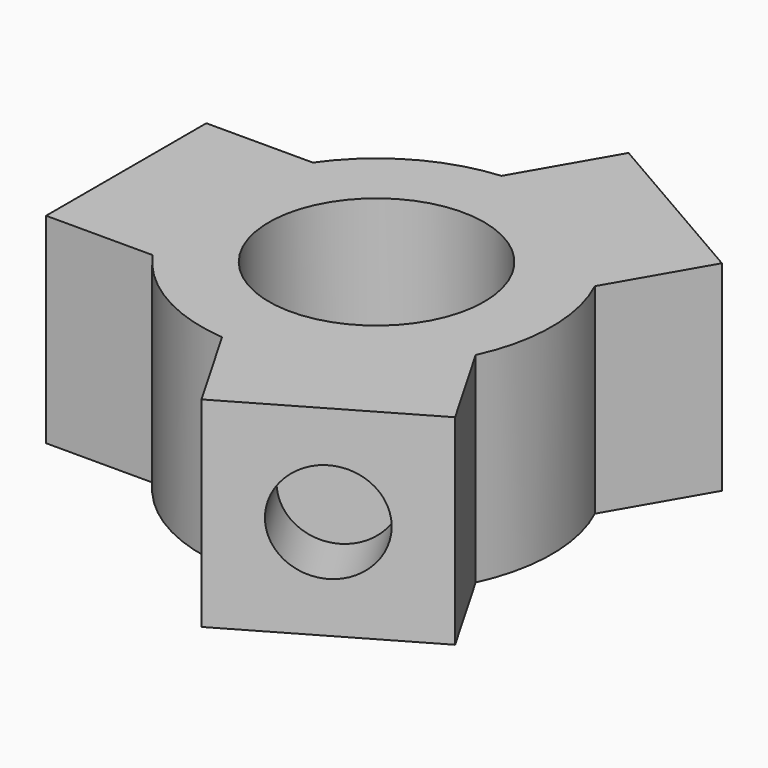
from build123d import *

# Parameters (mm, degrees)
F0_R     = 21.5
F1_DEPTH = 40
F2_R     = 10
F5_DEPTH = 12
F3_R     = 10
F6_DEPTH = 12
F4_R     = 10
F7_DEPTH = 12


# Not quite as in the source:
# - a feature names something its author has since deleted; it is built from what else it names


with BuildPart() as f1:
    # F0 (on Top) → F1 (new body)
    with BuildSketch(Plane.XY):
        with BuildLine():
            Line((7.6794919243, 53.3012701892), (-2.9591014593, 34.8746859277))
            ThreePointArc((-2.9591014593, 34.8746859277), (-17.5, 30.3108891325), (-28.7228132327, 20))
            Line((-28.7228132327, 20), (-50, 20))
            Line((-50, 20), (-50, -20))
            Line((-50, -20), (-28.7228132327, -20))
            ThreePointArc((-28.7228132327, -20), (-17.5, -30.3108891325), (-2.9591014593, -34.8746859277))
            Line((-2.9591014593, -34.8746859277), (7.6794919243, -53.3012701892))
            Line((7.6794919243, -53.3012701892), (42.3205080757, -33.3012701892))
            Line((42.3205080757, -33.3012701892), (31.681914692, -14.8746859277))
            ThreePointArc((31.681914692, -14.8746859277), (35, 0), (31.681914692, 14.8746859277))
            Line((31.681914692, 14.8746859277), (42.3205080757, 33.3012701892))
            Line((42.3205080757, 33.3012701892), (7.6794919243, 53.3012701892))
        make_face()
        Circle(F0_R, mode=Mode.SUBTRACT)
    extrude(amount=-F1_DEPTH)

    # F2 (on face) → F5 (cut)
    with BuildSketch(Plane(origin=(-50, 0, 0), x_dir=(0, -1, 0), z_dir=(-1, 0, 0))):
        with Locations((0, -20)):
            Circle(F2_R)
    extrude(amount=-F5_DEPTH, mode=Mode.SUBTRACT)

    # F3 (on face) → F6 (cut)
    with BuildSketch(Plane(origin=(25, -43.3012701892, 0), x_dir=(0.8660254038, 0.5, 0), z_dir=(0.5, -0.8660254038, 0))):
        with Locations((0, -20)):
            Circle(F3_R)
    extrude(amount=-F6_DEPTH, mode=Mode.SUBTRACT)

    # F4 (on face) → F7 (cut)
    with BuildSketch(Plane(origin=(25, 43.3012701892, 0), x_dir=(-0.8660254038, 0.5, 0), z_dir=(0.5, 0.8660254038, 0))):
        with Locations((0, -20)):
            Circle(F4_R)
    extrude(amount=-F7_DEPTH, mode=Mode.SUBTRACT)


solid = f1.part
